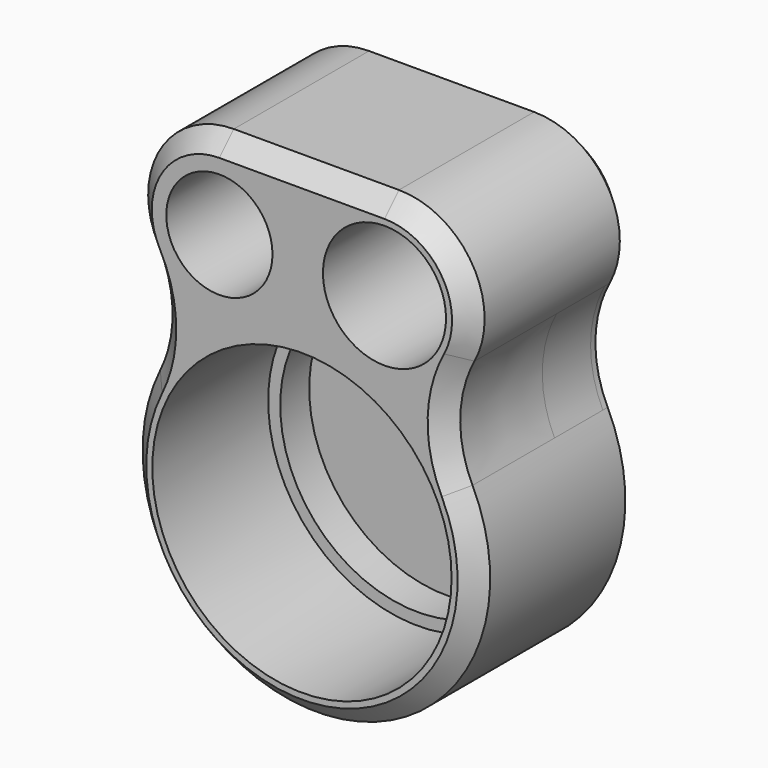
from build123d import *

# Parameters (mm, degrees)
F0_R     = 4.4
F1_DEPTH = 5
F2_DEPTH = 2
F3_R     = 10
F4_DEPTH = 3
F5_DEPTH = 4
F6_DEPTH = 10
F7_SIZE  = 1.5


with BuildPart() as f1:
    # F0 (on Front) → F1 (new body)
    with BuildSketch(Plane.XZ):
        with BuildLine():
            ThreePointArc((-5.4134613959, 11.1559148309), (4.2410497772, 11.6521884977), (11.3178358484, 5.0662206533))
            Line((11.3178358484, 5.0662206533), (11.2530788382, 8.9848882386))
            ThreePointArc((11.2530788382, 8.9848882386), (9.8365288611, 10.5167818254), (8.2134709888, 11.8278862996))
            ThreePointArc((8.2134709888, 11.8278862996), (9.7771968263, 12.3297019504), (11.1837970537, 13.1773653522))
            Line((11.1837970537, 13.1773653522), (11.1364032022, 16.0453289729))
            ThreePointArc((11.1364032022, 16.0453289729), (5.0961001356, 14.0014200497), (1.7827588677, 19.4497770926))
            Line((1.7827588677, 19.4497770926), (-5.4134613959, 11.1559148309))
        make_face()
        with BuildLine():
            ThreePointArc((11.3178358484, 5.0662206533), (12.1264414508, 2.5902543774), (12.4, 0))
            ThreePointArc((12.4, 0), (-6.5815301675, -10.5092083743), (-5.4134613959, 11.1559148309))
            Line((-5.4134613959, 11.1559148309), (1.7827588677, 19.4497770926))
            ThreePointArc((1.7827588677, 19.4497770926), (7.1690482729, 23.8832523997), (11.9404028665, 18.7938524157))
            ThreePointArc((11.9404028665, 18.7938524157), (11.7352778247, 17.362000767), (11.1364032022, 16.0453289729))
            Line((11.1364032022, 16.0453289729), (11.1837970537, 13.1773653522))
            ThreePointArc((11.1837970537, 13.1773653522), (13.5592963078, 21.0887316989), (6.8404028665, 25.8938524157))
            Line((6.8404028665, 25.8938524157), (-6.8404028665, 25.8938524157))
            ThreePointArc((-6.8404028665, 25.8938524157), (-13.9068149485, 19.4836496958), (-8.2134709888, 11.8278862996))
            ThreePointArc((-8.2134709888, 11.8278862996), (-2.0809765648, -14.2488433403), (11.2530788382, 8.9848882386))
            Line((11.2530788382, 8.9848882386), (11.3178358484, 5.0662206533))
        make_face()
        with Locations((-6.8404028665, 18.7938524157)):
            Circle(F0_R, mode=Mode.SUBTRACT)
    extrude(amount=F1_DEPTH)

    # F0 (on Front) → F2 (join)
    with BuildSketch(Plane.XZ):
        with BuildLine():
            ThreePointArc((11.3178358484, 5.0662206533), (12.1264414508, 2.5902543774), (12.4, 0))
            ThreePointArc((12.4, 0), (-6.5815301675, -10.5092083743), (-5.4134613959, 11.1559148309))
            Line((-5.4134613959, 11.1559148309), (1.7827588677, 19.4497770926))
            ThreePointArc((1.7827588677, 19.4497770926), (7.1690482729, 23.8832523997), (11.9404028665, 18.7938524157))
            ThreePointArc((11.9404028665, 18.7938524157), (11.7352778247, 17.362000767), (11.1364032022, 16.0453289729))
            Line((11.1364032022, 16.0453289729), (11.1837970537, 13.1773653522))
            ThreePointArc((11.1837970537, 13.1773653522), (13.5592963078, 21.0887316989), (6.8404028665, 25.8938524157))
            Line((6.8404028665, 25.8938524157), (-6.8404028665, 25.8938524157))
            ThreePointArc((-6.8404028665, 25.8938524157), (-13.9068149485, 19.4836496958), (-8.2134709888, 11.8278862996))
            ThreePointArc((-8.2134709888, 11.8278862996), (-2.0809765648, -14.2488433403), (11.2530788382, 8.9848882386))
            Line((11.2530788382, 8.9848882386), (11.3178358484, 5.0662206533))
        make_face()
        with Locations((-6.8404028665, 18.7938524157)):
            Circle(F0_R, mode=Mode.SUBTRACT)
        with BuildLine():
            ThreePointArc((-5.4134613959, 11.1559148309), (4.2410497772, 11.6521884977), (11.3178358484, 5.0662206533))
            Line((11.3178358484, 5.0662206533), (11.2530788382, 8.9848882386))
            ThreePointArc((11.2530788382, 8.9848882386), (9.8365288611, 10.5167818254), (8.2134709888, 11.8278862996))
            ThreePointArc((8.2134709888, 11.8278862996), (9.7771968263, 12.3297019504), (11.1837970537, 13.1773653522))
            Line((11.1837970537, 13.1773653522), (11.1364032022, 16.0453289729))
            ThreePointArc((11.1364032022, 16.0453289729), (5.0961001356, 14.0014200497), (1.7827588677, 19.4497770926))
            Line((1.7827588677, 19.4497770926), (-5.4134613959, 11.1559148309))
        make_face()
        with BuildLine():
            ThreePointArc((11.0898226812, 18.8640751933), (8.2939884756, 22.7875460541), (3.6302967624, 21.5791205895))
            ThreePointArc((3.6302967624, 21.5791205895), (5.3538718279, 14.8123042908), (11.0904028665, 18.7938524157))
            ThreePointArc((11.0904028665, 18.7938524157), (11.0902578177, 18.8289650029), (11.0898226812, 18.8640751933))
        make_face()
        with BuildLine():
            Line((3.6302967624, 21.5791205895), (1.7827588677, 19.4497770926))
            ThreePointArc((1.7827588677, 19.4497770926), (5.0961001356, 14.0014200497), (11.1364032022, 16.0453289729))
            Line((11.1364032022, 16.0453289729), (11.0898226812, 18.8640751933))
            ThreePointArc((11.0898226812, 18.8640751933), (11.0902578177, 18.8289650029), (11.0904028665, 18.7938524157))
            ThreePointArc((11.0904028665, 18.7938524157), (5.3538718279, 14.8123042908), (3.6302967624, 21.5791205895))
        make_face()
        with BuildLine():
            ThreePointArc((11.9404028665, 18.7938524157), (7.1690482729, 23.8832523997), (1.7827588677, 19.4497770926))
            Line((1.7827588677, 19.4497770926), (3.6302967624, 21.5791205895))
            ThreePointArc((3.6302967624, 21.5791205895), (8.2939884756, 22.7875460541), (11.0898226812, 18.8640751933))
            Line((11.0898226812, 18.8640751933), (11.1364032022, 16.0453289729))
            ThreePointArc((11.1364032022, 16.0453289729), (11.7352778247, 17.362000767), (11.9404028665, 18.7938524157))
        make_face()
        with BuildLine():
            Line((11.3984437382, 0.188362274), (11.3178358484, 5.0662206533))
            ThreePointArc((11.3178358484, 5.0662206533), (4.2410497772, 11.6521884977), (-5.4134613959, 11.1559148309))
            Line((-5.4134613959, 11.1559148309), (-8.61063755, 7.471072278))
            ThreePointArc((-8.61063755, 7.471072278), (-3.8990296339, -10.712495877), (11.3984437382, 0.188362274))
        make_face()
        with BuildLine():
            ThreePointArc((-5.4134613959, 11.1559148309), (-6.5815301675, -10.5092083743), (12.4, 0))
            ThreePointArc((12.4, 0), (12.1264414508, 2.5902543774), (11.3178358484, 5.0662206533))
            Line((11.3178358484, 5.0662206533), (11.3984437382, 0.188362274))
            ThreePointArc((11.3984437382, 0.188362274), (-3.8990296339, -10.712495877), (-8.61063755, 7.471072278))
            Line((-8.61063755, 7.471072278), (-5.4134613959, 11.1559148309))
        make_face()
    extrude(amount=-F2_DEPTH)

    # F3
    f3_edges = [f1.edges().sort_by_distance(p)[0] for p in [
        (8.213471, -1.5, 11.827886),
        (-8.213471, -1.5, 11.827886),
    ]]
    fillet(f3_edges, radius=F3_R)

    # F0 (on Front) → F4 (join)
    with BuildSketch(Plane.XZ):
        with BuildLine():
            ThreePointArc((-5.4134613959, 11.1559148309), (-6.5815301675, -10.5092083743), (12.4, 0))
            ThreePointArc((12.4, 0), (12.1264414508, 2.5902543774), (11.3178358484, 5.0662206533))
            Line((11.3178358484, 5.0662206533), (11.3984437382, 0.188362274))
            ThreePointArc((11.3984437382, 0.188362274), (-3.8990296339, -10.712495877), (-8.61063755, 7.471072278))
            Line((-8.61063755, 7.471072278), (-5.4134613959, 11.1559148309))
        make_face()
        with BuildLine():
            ThreePointArc((11.9404028665, 18.7938524157), (7.1690482729, 23.8832523997), (1.7827588677, 19.4497770926))
            Line((1.7827588677, 19.4497770926), (3.6302967624, 21.5791205895))
            ThreePointArc((3.6302967624, 21.5791205895), (8.2939884756, 22.7875460541), (11.0898226812, 18.8640751933))
            Line((11.0898226812, 18.8640751933), (11.1364032022, 16.0453289729))
            ThreePointArc((11.1364032022, 16.0453289729), (11.7352778247, 17.362000767), (11.9404028665, 18.7938524157))
        make_face()
    extrude(amount=F4_DEPTH)

    # F0 (on Front) → F5 (cut)
    with BuildSketch(Plane.XZ):
        with BuildLine():
            Line((11.3984437382, 0.188362274), (11.3178358484, 5.0662206533))
            ThreePointArc((11.3178358484, 5.0662206533), (4.2410497772, 11.6521884977), (-5.4134613959, 11.1559148309))
            Line((-5.4134613959, 11.1559148309), (-8.61063755, 7.471072278))
            ThreePointArc((-8.61063755, 7.471072278), (-3.8990296339, -10.712495877), (11.3984437382, 0.188362274))
        make_face()
        with BuildLine():
            ThreePointArc((-5.4134613959, 11.1559148309), (4.2410497772, 11.6521884977), (11.3178358484, 5.0662206533))
            Line((11.3178358484, 5.0662206533), (11.2530788382, 8.9848882386))
            ThreePointArc((11.2530788382, 8.9848882386), (9.8365288611, 10.5167818254), (8.2134709888, 11.8278862996))
            ThreePointArc((8.2134709888, 11.8278862996), (9.7771968263, 12.3297019504), (11.1837970537, 13.1773653522))
            Line((11.1837970537, 13.1773653522), (11.1364032022, 16.0453289729))
            ThreePointArc((11.1364032022, 16.0453289729), (5.0961001356, 14.0014200497), (1.7827588677, 19.4497770926))
            Line((1.7827588677, 19.4497770926), (-5.4134613959, 11.1559148309))
        make_face()
        with BuildLine():
            Line((3.6302967624, 21.5791205895), (1.7827588677, 19.4497770926))
            ThreePointArc((1.7827588677, 19.4497770926), (5.0961001356, 14.0014200497), (11.1364032022, 16.0453289729))
            Line((11.1364032022, 16.0453289729), (11.0898226812, 18.8640751933))
            ThreePointArc((11.0898226812, 18.8640751933), (11.0902578177, 18.8289650029), (11.0904028665, 18.7938524157))
            ThreePointArc((11.0904028665, 18.7938524157), (5.3538718279, 14.8123042908), (3.6302967624, 21.5791205895))
        make_face()
        with BuildLine():
            ThreePointArc((11.0898226812, 18.8640751933), (8.2939884756, 22.7875460541), (3.6302967624, 21.5791205895))
            ThreePointArc((3.6302967624, 21.5791205895), (5.3538718279, 14.8123042908), (11.0904028665, 18.7938524157))
            ThreePointArc((11.0904028665, 18.7938524157), (11.0902578177, 18.8289650029), (11.0898226812, 18.8640751933))
        make_face()
        with BuildLine():
            ThreePointArc((8.2134709888, 11.8278862996), (9.8365288611, 10.5167818254), (11.2530788382, 8.9848882386))
            Line((11.2530788382, 8.9848882386), (11.1837970537, 13.1773653522))
            ThreePointArc((11.1837970537, 13.1773653522), (9.7771968263, 12.3297019504), (8.2134709888, 11.8278862996))
        make_face()
    extrude(amount=F5_DEPTH, mode=Mode.SUBTRACT)

    # F6 (add): a face of the model
    f6_faces = [f1.faces().sort_by_distance(p)[0] for p in [
        (12.5064069452, -5, 22.1877746808),
    ]]
    extrude(f6_faces, amount=F6_DEPTH)

    # F7
    f7_edges = [f1.edges().sort_by_distance(p)[0] for p in [
        (0, 2, -14.4),
        (0, -15, -14.4),
        (12.931295, -15, 22.442281),
        (12.931295, 2, 22.442281),
        (-11.918405, 2, 10.906319),
        (11.918405, 2, 10.906319),
        (-12.931295, 2, 22.442281),
        (0, 2, 25.893852),
        (-12.931295, -15, 22.442281),
        (-11.918405, -15, 10.906319),
        (0, -15, 25.893852),
        (11.918405, -15, 10.906319),
    ]]
    chamfer(f7_edges, length=F7_SIZE)


solid = f1.part
